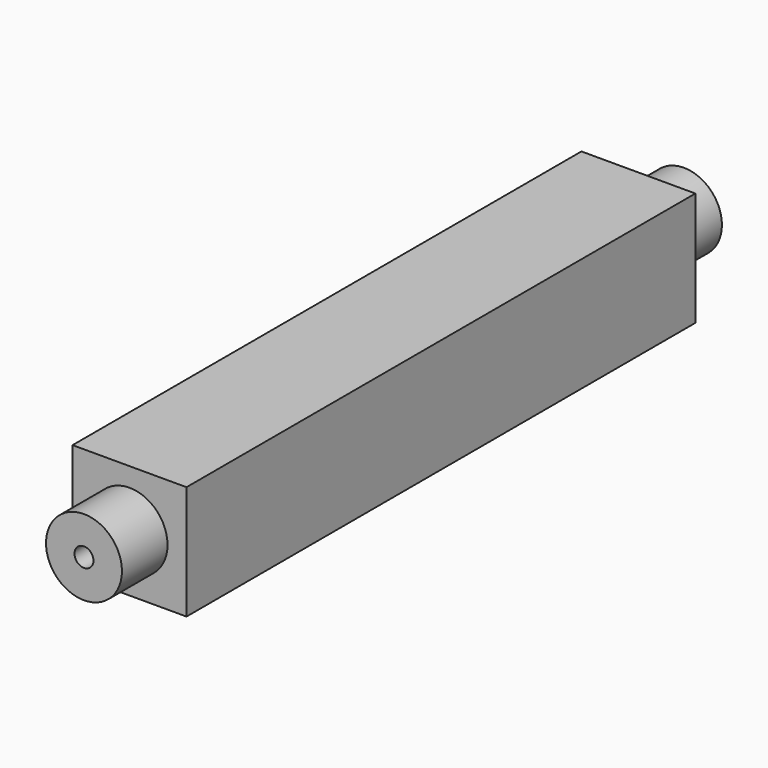
from build123d import *

# Parameters (mm, degrees)
F0_R     = 2
F1_DEPTH = 3
F2_W     = 6
F2_H     = 6
F2_R     = 2
F3_DEPTH = 33.5
F4_DEPTH = 36.5
F5_R     = 0.5
F6_DEPTH = 5
F7_R     = 0.5
F8_DEPTH = 5


with BuildPart() as f1:
    # F0 (on Front) → F1 (new body)
    with BuildSketch(Plane.XZ):
        Circle(F0_R)
    extrude(amount=F1_DEPTH)


with BuildPart() as f3:
    # F2 (on face) → F3 (new body)
    with BuildSketch(Plane.XZ.offset(3)):
        Rectangle(F2_W, F2_H)
        Circle(F2_R, mode=Mode.SUBTRACT)
    extrude(amount=F3_DEPTH)


with BuildPart() as f4:
    # F4 (new): a face of the model
    f4_faces = [f1.part.faces().sort_by_distance(p)[0] for p in [
        (0, -3, 0),
    ]]
    extrude(f4_faces, amount=F4_DEPTH)

    # F5 (on face) → F6 (cut)
    with BuildSketch(Plane.XZ.offset(39.5)):
        Circle(F5_R)
    extrude(amount=-F6_DEPTH, mode=Mode.SUBTRACT)


with BuildPart() as f1_1:
    add(f1.part)

    # F7 (on face) → F8 (cut)
    with BuildSketch(Plane(origin=(0, 0, 0), x_dir=(-1, 0, 0), z_dir=(0, 1, 0))):
        Circle(F7_R)
    extrude(amount=-F8_DEPTH, mode=Mode.SUBTRACT)


solid = Compound([f3.part, f4.part, f1_1.part])
